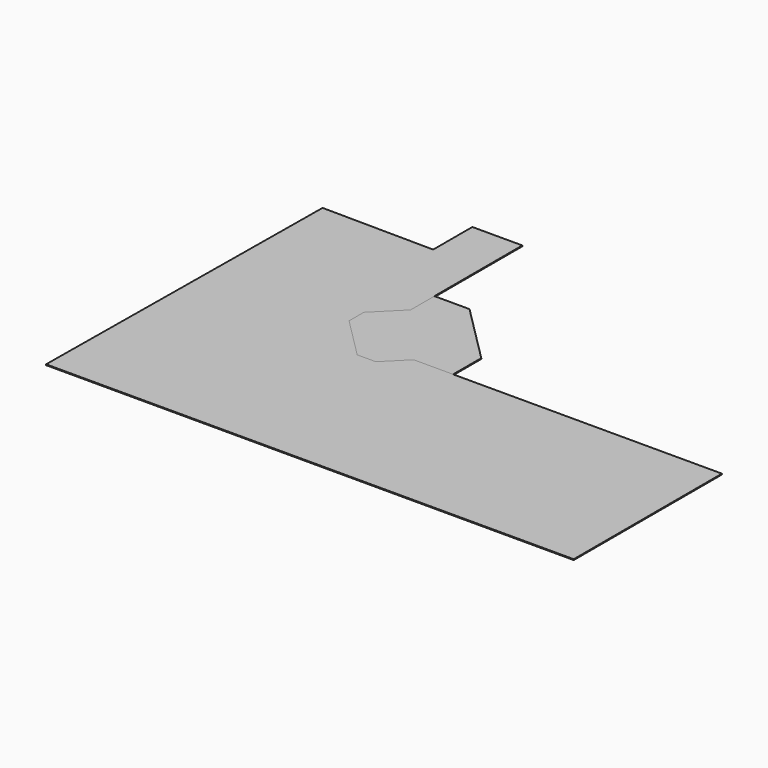
from build123d import *

# Parameters (mm, degrees)
F1_DEPTH = 25
F2_DEPTH = 25


# Not quite as in the source:
# - the program builds the solid bodies; features that only make, move or delete a surface that nothing else refers to are left out


with BuildPart() as f1:
    # F3 (on Top) → F1 (new body)
    with BuildSketch(Plane.XY):
        Polygon((-131.7934449173, 9299.8765415886), (-234.5616734816, -1019.6117544074), (15715.4383265184, -1019.6117544074), (15715.4383265184, 4580.3882455926), (7589.948546532, 4580.3882455926), (6396.9839009692, 4580.3882455926), (5760.5877979013, 3943.9921425247), (5200.5877979013, 3943.9921425247), (3963.1509308248, 5181.4290096012), (3963.1509308248, 5741.4290096012), (4748.0394579419, 6526.3175367182), (4748.0394579419, 7426.3175367182), (4748.0394579419, 10746.3175367182), (3238.0394579419, 10746.3175367182), (3238.0394579419, 9266.3175367182), align=None)
    extrude(amount=F1_DEPTH)


with BuildPart() as f2:
    # F3 (on Top) → F2 (new body)
    with BuildSketch(Plane.XY):
        Polygon((6396.9839009692, 4580.3882455926), (7589.948546532, 4580.3882455926), (7589.948546532, 5644.4084481281), (5808.0394579419, 7426.3175367182), (4748.0394579419, 7426.3175367182), (4748.0394579419, 6526.3175367182), (3963.1509308248, 5741.4290096012), (3963.1509308248, 5181.4290096012), (5200.5877979013, 3943.9921425247), (5760.5877979013, 3943.9921425247), align=None)
    extrude(amount=F2_DEPTH)


solid = Compound([f1.part, f2.part])
